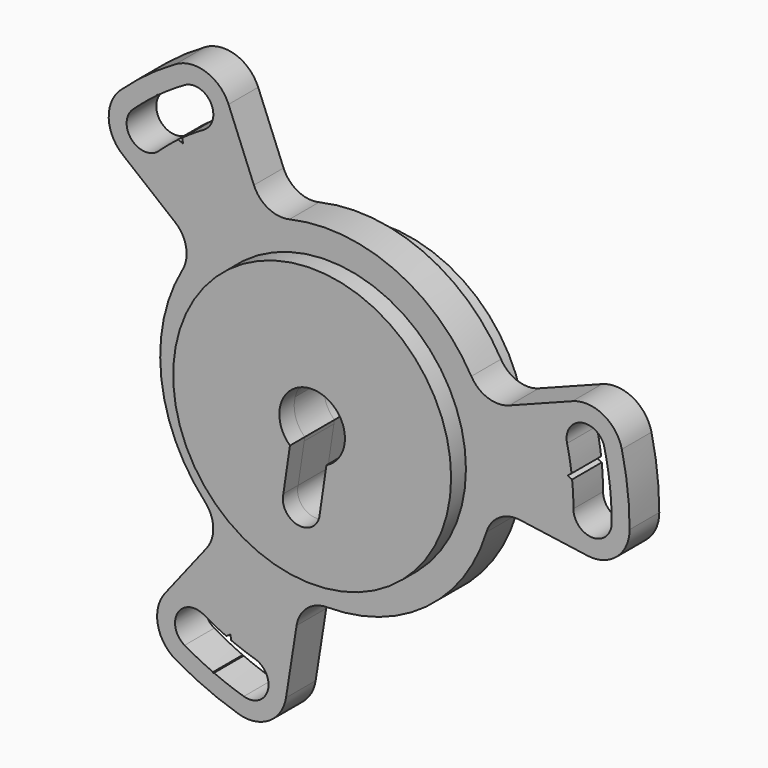
from build123d import *
from build123d import SkipClean  # not in build123d's __all__

# Parameters (mm, degrees)
F1_DEPTH      = 6
F2_R          = 22.5
F3_DEPTH      = 3
F3_DEPTH_BACK = 12


with BuildPart() as f1:
    # F0 (on Front) → F1 (new body)
    with BuildSketch(Plane.XZ):
        with BuildLine():
            ThreePointArc((-15.9360760742, 39.4846993069), (-19.545554777, 42.911846885), (-24.5, 42.4352447854))
            ThreePointArc((-24.5, 42.4352447854), (-29.1533569815, 39.3837755518), (-33.430729205, 35.824381988))
            ThreePointArc((-33.430729205, 35.824381988), (-35.3334015022, 31.2250869161), (-33.1097213112, 26.7721189803))
            Line((-33.1097213112, 26.7721189803), (-24.5775940866, 19.8731444143))
            ThreePointArc((-24.5775940866, 19.8731444143), (-22.8056864044, 16.8994131973), (-23.3899197808, 13.487462795))
            ThreePointArc((-23.3899197808, 13.487462795), (-26.8258933187, -3.0612820274), (-19.7498381023, -18.410428972))
            ThreePointArc((-19.7498381023, -18.410428972), (-18.4119152904, -21.6030292813), (-19.4682866758, -24.8995143308))
            Line((-19.4682866758, -24.8995143308), (-26.2267146235, -33.5433963703))
            ThreePointArc((-26.2267146235, -33.5433963703), (-27.3899721372, -38.3828704105), (-24.5, -42.4352447854))
            ThreePointArc((-24.5, -42.4352447854), (-19.530671634, -44.9394355274), (-14.3094602739, -46.8640517526))
            ThreePointArc((-14.3094602739, -46.8640517526), (-9.3750177536, -46.212166761), (-6.6304744945, -42.0599192579))
            Line((-6.6304744945, -42.0599192579), (-4.9218508726, -31.2213930501))
            ThreePointArc((-4.9218508726, -31.2213930501), (-3.2324779357, -28.2000103756), (0.0144744773, -26.9999961202))
            ThreePointArc((0.0144744773, -26.9999961202), (16.0640946633, -21.7012640795), (25.8188182355, -7.8986470313))
            ThreePointArc((25.8188182355, -7.8986470313), (27.9147298015, -5.1436717332), (31.2977552903, -4.410273664))
            Line((31.2977552903, -4.410273664), (42.1627906977, -5.9413029366))
            ThreePointArc((42.1627906977, -5.9413029366), (46.9355269143, -4.5289764745), (49, 0))
            ThreePointArc((49, 0), (48.6840286155, 5.5556599757), (47.740189479, 11.0396697646))
            ThreePointArc((47.740189479, 11.0396697646), (44.7084192558, 14.987079845), (39.7401958057, 15.2878002776))
            Line((39.7401958057, 15.2878002776), (29.4994449592, 11.3482486357))
            ThreePointArc((29.4994449592, 11.3482486357), (26.0381643401, 11.3005971783), (23.3754453035, 13.5125333252))
            ThreePointArc((23.3754453035, 13.5125333252), (10.7617986555, 24.7625461069), (-6.0689801331, 26.3090760032))
            ThreePointArc((-6.0689801331, 26.3090760032), (-9.5028145111, 26.7467010144), (-11.8294686145, 29.3097879948))
            Line((-11.8294686145, 29.3097879948), (-15.9360760742, 39.4846993069))
        make_face()
        with BuildLine():
            ThreePointArc((-18.2977896407, -42.3131291004), (-18.3599561093, -42.3518337374), (-18.4225903326, -42.3897767579))
            ThreePointArc((-18.4225903326, -42.3897767579), (-18.4375826284, -42.3180972643), (-18.4516989687, -42.2462401305))
            ThreePointArc((-18.4516989687, -42.2462401305), (-20.7833159026, -41.1492865077), (-23.05, -39.9237711145))
            ThreePointArc((-23.05, -39.9237711145), (-24.1846787517, -35.6890923627), (-19.95, -34.554413611))
            ThreePointArc((-19.95, -34.554413611), (-18.1421434856, -35.5369192496), (-16.2860412235, -36.4249208821))
            ThreePointArc((-16.2860412235, -36.4249208821), (-15.9677964631, -36.1891617461), (-15.6346911323, -35.9749120408))
            ThreePointArc((-15.6346911323, -35.9749120408), (-15.5640668297, -36.3646225815), (-15.519307053, -36.7581434324))
            ThreePointArc((-15.519307053, -36.7581434324), (-13.6037364042, -37.5093102555), (-11.6519890802, -38.1607278557))
            ThreePointArc((-11.6519890802, -38.1607278557), (-9.5924128846, -42.0308888206), (-13.4625738495, -44.0904650162))
            ThreePointArc((-13.4625738495, -44.0904650162), (-15.9050276013, -43.2693898386), (-18.2977896407, -42.3131291004))
        make_face(mode=Mode.SUBTRACT)
        with BuildLine():
            ThreePointArc((2.0410607887, 4.9020578186), (3.3561252192, 4.1149147638), (4.3915942436, 2.9849623113))
            ThreePointArc((4.3915942436, 2.9849623113), (5.3099999882, 0.0003538209), (4.3919919982, -2.9843770351))
            ThreePointArc((4.3919919982, -2.9843770351), (3.4698827698, -4.0194543864), (2.3112879445, -4.7805907624))
            Line((2.3112879445, -4.7805907624), (1.2434795246, -12.010568624))
            ThreePointArc((1.2434795246, -12.010568624), (-2.1944705259, -14.838607263), (-4.6609590448, -11.1327015059))
            Line((-4.6609590448, -11.1327015059), (-3.6838317901, -4.5167128251))
            Line((-3.6838317901, -4.5167128251), (-3.5940513986, -3.9088226545))
            ThreePointArc((-3.5940513986, -3.9088226545), (-5.0887135619, -1.5169358209), (-5.1476659417, 1.3029333647))
            ThreePointArc((-5.1476659417, 1.3029333647), (-4.6350123617, 2.5908995362), (-3.8064652091, 3.7022861332))
            ThreePointArc((-3.8064652091, 3.7022861332), (-1.0672517117, 5.2016414509), (2.0410607887, 4.9020578186))
        make_face(mode=Mode.SUBTRACT)
        with BuildLine():
            ThreePointArc((-23.05, 39.9237711145), (-18.8153212483, 38.7890923627), (-19.95, 34.554413611))
            ThreePointArc((-19.95, 34.554413611), (-21.7048030996, 33.4800167624), (-23.401886203, 32.3165858677))
            ThreePointArc((-23.401886203, 32.3165858677), (-23.3568351823, 31.9230982526), (-23.3378421601, 31.5274957213))
            ThreePointArc((-23.3378421601, 31.5274957213), (-23.7106535397, 31.6611885515), (-24.0738324819, 31.8191858732))
            ThreePointArc((-24.0738324819, 31.8191858732), (-25.6821473576, 30.5358364402), (-27.2221652098, 29.1712824759))
            ThreePointArc((-27.2221652098, 29.1712824759), (-31.60361102, 29.322717652), (-31.4521758439, 33.7041634621))
            ThreePointArc((-31.4521758439, 33.7041634621), (-29.5198770058, 35.4088528699), (-27.4953498942, 37.0029152121))
            ThreePointArc((-27.4953498942, 37.0029152121), (-27.4977858588, 37.0761052717), (-27.4993283668, 37.1493196105))
            ThreePointArc((-27.4993283668, 37.1493196105), (-27.4297559565, 37.1264635728), (-27.3604676831, 37.1027601152))
            ThreePointArc((-27.3604676831, 37.1027601152), (-25.244669512, 38.5735228004), (-23.05, 39.9237711145))
        make_face(mode=Mode.SUBTRACT)
        with BuildLine():
            ThreePointArc((45.7931395349, 5.3102138882), (45.8577419681, 5.2757284657), (45.9219186994, 5.2404571474))
            ThreePointArc((45.9219186994, 5.2404571474), (45.8673385849, 5.1916336916), (45.8121666518, 5.1434800154))
            ThreePointArc((45.8121666518, 5.1434800154), (46.0279854146, 2.5757637074), (46.1, 0))
            ThreePointArc((46.1, 0), (43, -3.1), (39.9, 0))
            ThreePointArc((39.9, 0), (39.8469465851, 2.0569024872), (39.6879274265, 4.1083350144))
            ThreePointArc((39.6879274265, 4.1083350144), (39.3246316454, 4.2660634935), (38.9725332924, 4.4474163195))
            ThreePointArc((38.9725332924, 4.4474163195), (39.2747203695, 4.70343403), (39.5931395349, 4.9389575592))
            ThreePointArc((39.5931395349, 4.9389575592), (39.2858837618, 6.9734738153), (38.87415429, 8.9894453798))
            ThreePointArc((38.87415429, 8.9894453798), (41.1960239046, 12.7081711687), (44.9147496935, 10.3863015541))
            ThreePointArc((44.9147496935, 10.3863015541), (45.4249046071, 7.8605369687), (45.7931395349, 5.3102138882))
        make_face(mode=Mode.SUBTRACT)
    extrude(amount=F1_DEPTH)

    # F2 (on face) → F3 (join, two sides)
    with BuildSketch(Plane.XZ.offset(6)) as f3_sk:
        Circle(F2_R)
        with BuildLine():
            Line((-4.6609590448, -11.1327015059), (-3.5940513986, -3.9088226545))
            ThreePointArc((-3.5940513986, -3.9088226545), (0.7754775485, 5.2530690621), (2.3112879445, -4.7805907624))
            Line((2.3112879445, -4.7805907624), (1.2434795246, -12.010568624))
            ThreePointArc((1.2434795246, -12.010568624), (-2.1944705259, -14.838607263), (-4.6609590448, -11.1327015059))
        make_face(mode=Mode.SUBTRACT)
    with SkipClean():  # cleaning this boolean's faces spoils the solid; the shape is the same uncleaned
        extrude(amount=F3_DEPTH)
        extrude(f3_sk.sketch, amount=-F3_DEPTH_BACK)


solid = f1.part
